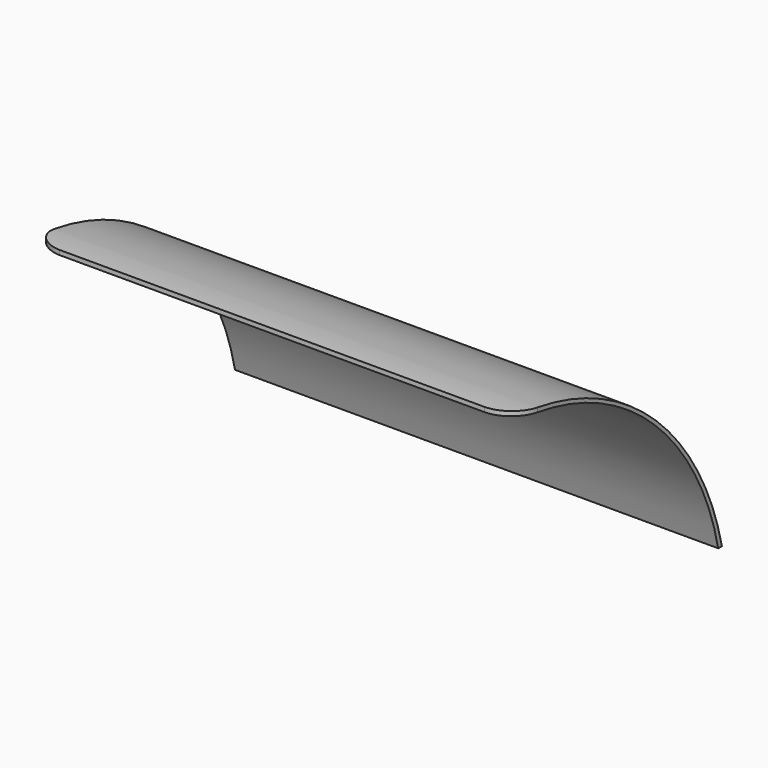
from build123d import *

# Parameters (mm, degrees)
F1_DEPTH      = 147.193
F1_DEPTH_BACK = 147.193
F3_DEPTH      = 186.182


# Not quite as in the source:
# - a length typed as a fraction of an inch, garbled in the dataset ("3 / 203.2 mm" for 3/8 in), is restored


with BuildPart() as f1:
    # F0 (on Right) → F1 (new body, two sides)
    with BuildSketch(Plane.YZ) as f1_sk:
        with BuildLine():
            ThreePointArc((-155.7030739649, 130.5633668295), (-55.3860759172, 92.0728226971), (0, 0))
            Line((0, 0), (2.794, 0))
            ThreePointArc((2.794, 0), (-53.8777768496, 93.5114749264), (-155.7030739649, 133.3573668295))
            Line((-155.7030739649, 133.3573668295), (-155.7030739649, 130.5633668295))
        make_face()
    extrude(amount=-F1_DEPTH)
    extrude(f1_sk.sketch, amount=F1_DEPTH_BACK)

    # F2 (on Top) → F3 (cut)
    with BuildSketch(Plane.XY):
        with BuildLine():
            ThreePointArc((-128.6797374487, -155.7030739649), (-141.8112510122, -150.4712953815), (-147.193, -137.4005290135))
            Line((-147.193, -137.4005290135), (-161.3427400589, -137.4005290135))
            Line((-161.3427400589, -137.4005290135), (-161.3427400589, -161.3346251115))
            Line((-161.3427400589, -161.3346251115), (-129.2428970337, -161.3346251115))
            Line((-129.2428970337, -161.3346251115), (-128.6797374487, -155.7030739649))
        make_face()
        with BuildLine():
            Line((128.6797374487, -155.7030739649), (129.2428970337, -161.3346251115))
            Line((129.2428970337, -161.3346251115), (161.3427400589, -161.3346251115))
            Line((161.3427400589, -161.3346251115), (161.3427400589, -137.4005290135))
            Line((161.3427400589, -137.4005290135), (147.193, -137.4005290135))
            ThreePointArc((147.193, -137.4005290135), (141.8112510122, -150.4712953815), (128.6797374487, -155.7030739649))
        make_face()
    extrude(amount=F3_DEPTH, mode=Mode.SUBTRACT)


solid = f1.part
